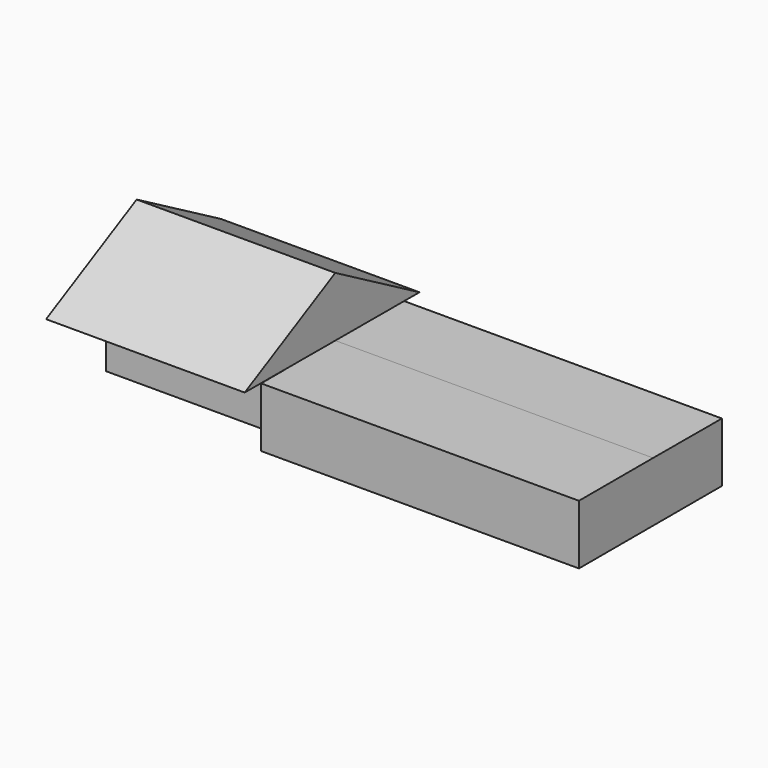
from build123d import *

# Parameters (mm, degrees)
F1_DEPTH = 16000
F2_W     = 7500
F2_H     = 3000
F3_DEPTH = 9000
F5_DEPTH = 10000


# Not quite as in the source:
# - the program builds the solid bodies; features that only make, move or delete a surface that nothing else refers to are left out


with BuildPart() as f1:
    # F0 (on Right) → F1 (new body)
    with BuildSketch(Plane.YZ):
        Polygon((4596.1385421307, 2968.7440507114), (-73.3513906598, 2968.7440507114), (-73.3513906598, -31.2559492886), (8926.6486093402, -31.2559492886), (8926.6486093402, 2957.9849909845), align=None)
    extrude(amount=F1_DEPTH)

    # F2 (on face) → F3 (join)
    with BuildSketch(Plane(origin=(0, 0, 0), x_dir=(0, -1, 0), z_dir=(-1, 0, 0))):
        with Locations((-5176.6486093402, 1468.7440507114)):
            Rectangle(F2_W, F2_H)
    extrude(amount=F3_DEPTH)

    # F0 (on Right) → F5 (join)
    with BuildSketch(Plane.YZ):
        Polygon((-1105.8957576752, 2982.9106330872), (4596.1385421307, 2968.7440507114), (8926.6486093402, 2968.7440507114), (8926.6486093402, 2957.9849909845), (9894.0702929946, 2955.5814524835), (4593.083292274, 5968.7609003512), align=None)
    extrude(amount=-F5_DEPTH)


solid = f1.part
